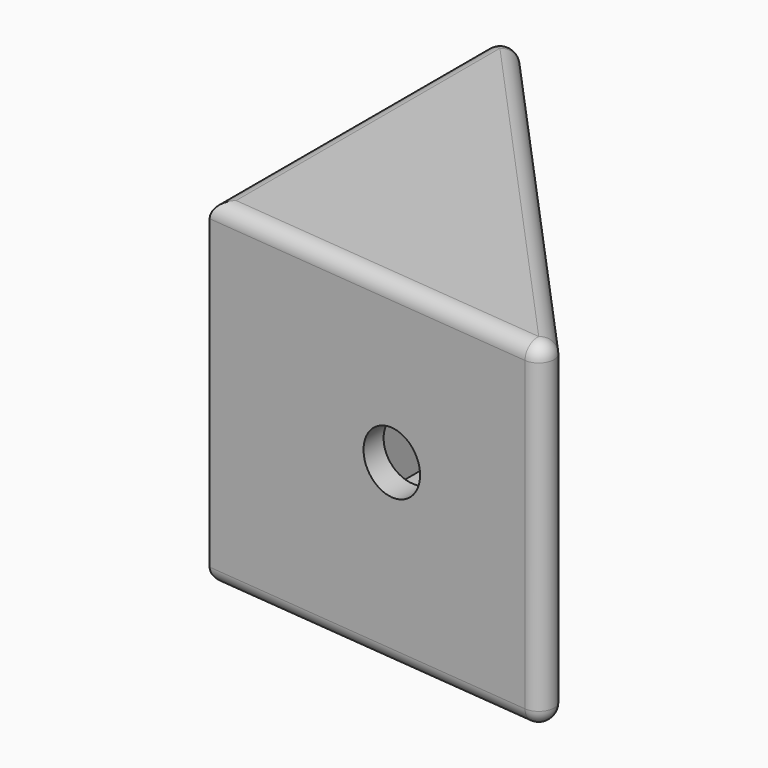
from build123d import *

# Parameters (mm, degrees)
F1_DEPTH     = 22
F2_R         = 1
F3_T1_DEPTH  = 31.8493182741
F3_T3_DEPTH  = 27.4759989859
F3_T8_DEPTH  = 1
F3_T14_DEPTH = 1
F4_R         = 1
F6_W         = 20.563358571
F6_H         = 20
F7_DEPTH     = 25
F9_D         = 4


# Not quite as in the source:
# - a fillet or chamfer that OpenCascade refuses, or shapes differently, is made with other operations: its cross-section is extruded or revolved along the edge and cut away or added


with BuildPart() as f1:
    # F0 (on Top) → F1 (new body)
    with BuildSketch(Plane.XY):
        Polygon((-24.8821492983, 2.4245919862), (0, 0), (-24.8821492983, 27.4245919862), align=None)
    extrude(amount=F1_DEPTH)

    # F2
    f2_edges = [f1.edges().sort_by_distance(p)[0] for p in [
        (-24.882149, 14.924592, 22),
        (-12.441075, 1.212296, 22),
    ]]
    fillet(f2_edges, radius=F2_R)

    # F3: fillet of radius 1 on 1 edges, made by hand

    # F3_s2 → F3_t1 (cut)
    with BuildSketch(Plane(origin=(-1.7406023493, 1.9184560251, 0), x_dir=(0, 0, 1), z_dir=(-0.6719435693, 0.7406023493, 0))):
        with BuildLine():
            ThreePointArc((21, 0), (21.7071067812, -0.2928932188), (22, -1))
            Line((22, -1), (22, 0))
            Line((22, 0), (21, 0))
        make_face()
    extrude(amount=F3_T1_DEPTH, mode=Mode.SUBTRACT)

    # F3_s4 → F3_t3 (cut)
    with BuildSketch(Plane.XY.offset(-6.4759989859)):
        with BuildLine():
            ThreePointArc((-24.8821492983, 24.8341923918), (-24.2422865296, 25.7670917297), (-23.141546949, 25.5061359611))
            Line((-23.141546949, 25.5061359611), (-24.8821492983, 27.4245919862))
            Line((-24.8821492983, 27.4245919862), (-24.8821492983, 24.8341923918))
        make_face()
        with BuildLine():
            ThreePointArc((-1.7406023493, 1.9184560251), (-1.5876305081, 0.7975969112), (-2.578188378, 0.2512264839))
            Line((-2.578188378, 0.2512264839), (0, 0))
            Line((0, 0), (-1.7406023493, 1.9184560251))
        make_face()
    extrude(amount=F3_T3_DEPTH, mode=Mode.SUBTRACT)


with BuildPart() as f3_tool6:
    # F3_s7 → F3_t8 (new body)
    with BuildSketch(Plane.XY.offset(21)):
        Polygon((-2.4812046985, 1.2465124558), (-1.7406023493, 1.9184560251), (0, 0), (-2.578188378, 0.2512264839), align=None)
    extrude(amount=F3_T8_DEPTH)

    # F3_s9 → F3_t10 (revolve, cut)
    with BuildSketch(Plane(origin=(-2.4812046985, 1.2465124558, 21), x_dir=(-0.8935741904, 0.4489155446, 0), z_dir=(0.4489155446, 0.8935741904, 0))):
        with BuildLine():
            ThreePointArc((0, -1), (1, 0), (0, 1))
            Line((0, 1), (0, -1))
        make_face()
    revolve(axis=Axis((-2.4812046985, 1.2465124558, 21), (0, 0, 1)), mode=Mode.SUBTRACT)


with BuildPart() as f1_1:
    add(f1.part)

    # F3_t5: cut F3_tool6
    add(f3_tool6.part, mode=Mode.SUBTRACT)


with BuildPart() as f3_tool12:
    # F3_s13 → F3_t14 (new body)
    with BuildSketch(Plane.XY.offset(21)):
        Polygon((-23.8821492983, 24.8341923918), (-24.8821492983, 24.8341923918), (-24.8821492983, 27.4245919862), (-23.141546949, 25.5061359611), align=None)
    extrude(amount=F3_T14_DEPTH)

    # F3_s15 → F3_t16 (revolve, cut)
    with BuildSketch(Plane(origin=(-23.8821492983, 24.8341923918, 21), x_dir=(0.3601372313, -0.9328993379, 0), z_dir=(-0.9328993379, -0.3601372313, 0))):
        with BuildLine():
            ThreePointArc((0, -1), (1, 0), (0, 1))
            Line((0, 1), (0, -1))
        make_face()
    revolve(axis=Axis((-23.8821492983, 24.8341923918, 21), (0, 0, 1)), mode=Mode.SUBTRACT)


with BuildPart() as f1_2:
    add(f1_1.part)

    # F3_t11: cut F3_tool12
    add(f3_tool12.part, mode=Mode.SUBTRACT)

    # F4
    f4_edges = [f1_2.edges().sort_by_distance(p)[0] for p in [
        (-13.730169, 1.337909, 0),
    ]]
    fillet(f4_edges, radius=F4_R)

    # F6 (on offset) → F7 (cut)
    with BuildSketch(Plane.XZ.offset(-3)):
        with Locations((-12.8598676635, 11)):
            Rectangle(F6_W, F6_H)
    extrude(amount=-F7_DEPTH, mode=Mode.SUBTRACT)

    # F9 (through all)
    with Locations(Plane(origin=(0, 3, 0), x_dir=(-1, 0, 0), z_dir=(0, 1, 0))):
        with Locations((12.000261806, 11.7051936686)):
            Hole(F9_D / 2)


solid = f1_2.part
